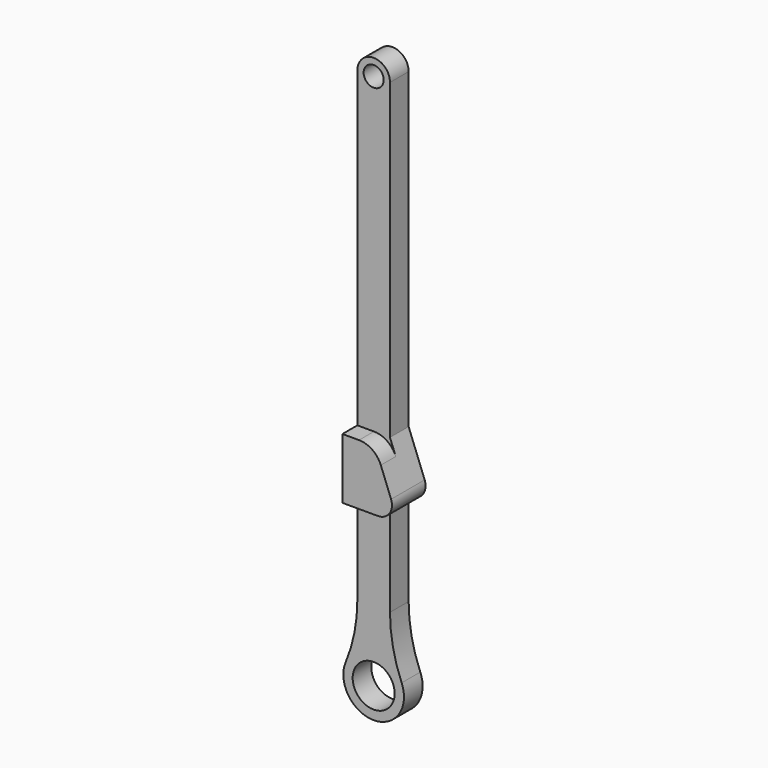
from build123d import *

# Parameters (mm, degrees)
F0_R          = 4.5
F0_R_2        = 2.15
F1_DEPTH      = 2.5
F3_DEPTH      = 4
F3_DEPTH_BACK = 5
F4_R          = 5
F5_R          = 3


with BuildPart() as f1:
    # F0 (on Front) → F1 (new body, symmetric)
    with BuildSketch(Plane.XZ):
        with BuildLine():
            ThreePointArc((-3.5, 15), (-4.13112804, 8.626225608), (-6, 2.5))
            ThreePointArc((-6, 2.5), (0, -6.5), (6, 2.5))
            ThreePointArc((6, 2.5), (4.13112804, 8.626225608), (3.5, 15))
            Line((3.5, 15), (3.5, 115))
            ThreePointArc((3.5, 115), (0, 118.5), (-3.5, 115))
            Line((-3.5, 115), (-3.5, 15))
        make_face()
        Circle(F0_R, mode=Mode.SUBTRACT)
        with Locations((0, 115)):
            Circle(F0_R_2, mode=Mode.SUBTRACT)
    extrude(amount=F1_DEPTH, both=True)

    # F2 (on face) → F3 (join, two sides)
    with BuildSketch(Plane.XZ.offset(2.5)) as f3_sk:
        Polygon((3.5, 48), (-3.5, 48), (-3.5, 35), (3.5, 35), (8.5, 35), align=None)
    extrude(amount=F3_DEPTH)
    extrude(f3_sk.sketch, amount=-F3_DEPTH_BACK)

    # F4
    f4_edges = [f1.edges().sort_by_distance(p)[0] for p in [
        (3.5, -4.5, 48),
    ]]
    fillet(f4_edges, radius=F4_R)

    # F5
    f5_edges = [f1.edges().sort_by_distance(p)[0] for p in [
        (8.5, -2, 35),
    ]]
    fillet(f5_edges, radius=F5_R)


solid = f1.part
